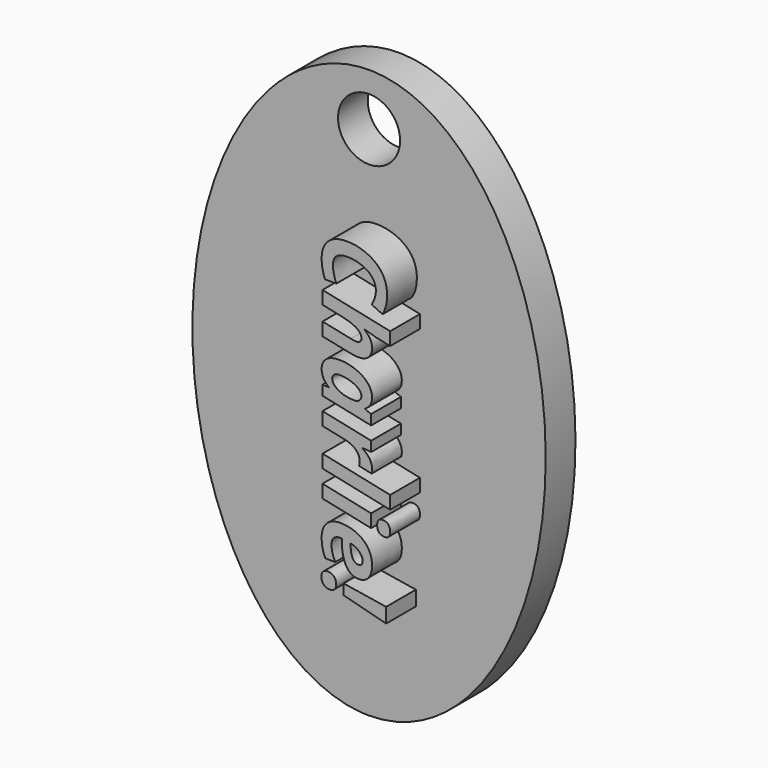
from build123d import *

# Parameters (mm, degrees)
F1_DEPTH     = 5
F2_R         = 4.1692191655
F3_DEPTH     = 5.0010001
F4_TEXT_SIZE = 11.9591396063
F5_DEPTH     = 5


# Not quite as in the source:
# - Text() gives the source's letters only with a copy of the font that has no kerning and outlines rounded to 1/6400 em; it was checked with that copy


with BuildPart() as f1:
    # F0 (on Front) → F1 (new body)
    with BuildSketch(Plane.XZ):
        with BuildLine():
            add(Edge.make_bspline(
                [(0, 0), (41.1089266517, 0), (20.5544633259, 57.2852678597), (0, 114.5705357194), (-20.5544633259, 57.2852678597), (-41.1089266517, 0), (0, 0)],
                knots=[0, 0, 0, 2.0943951024, 2.0943951024, 4.1887902048, 4.1887902048, 6.2831853072, 6.2831853072, 6.2831853072], degree=2, weights=[1, 0.5, 1, 0.5, 1, 0.5, 1]))
        make_face()
    extrude(amount=F1_DEPTH)

    # F2 (on face) → F3 (cut, through all)
    with BuildSketch(Plane.XZ.offset(5)):
        with Locations((0, 69.3487823009)):
            Circle(F2_R)
    extrude(amount=-F3_DEPTH, mode=Mode.SUBTRACT)

    # F4 (on face) → F5 (join)
    with BuildSketch(Plane.XZ.offset(5)):
        with Locations(Location((-2.25, 59.1795631355), (0, 0, -90))):
            Text('Charlie!', F4_TEXT_SIZE, font='Open Sans', font_style=FontStyle.BOLDITALIC, text_align=(TextAlign.LEFT, TextAlign.BOTTOM))
    extrude(amount=F5_DEPTH)


solid = f1.part
